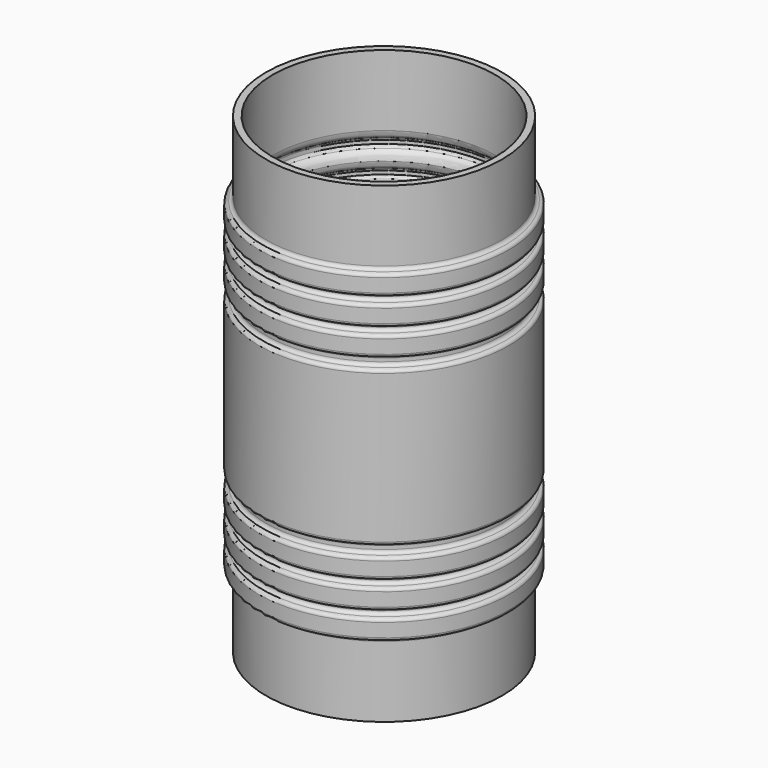
from build123d import *


# Not quite as in the source:
# - ends of sketch curves that miss each other by under 0.0002 mm in the source are joined


with BuildPart() as f1:
    # F0 (on Front) → F1 (revolve)
    with BuildSketch(Plane.XZ):
        with BuildLine():
            Line((-3.5, 2), (-3.5, 0))
            Line((-3.5, 0), (-3.3, 0))
            Line((-3.3, 0), (-3.3, 2.1))
            ThreePointArc((-3.3, 2.1), (-3.3401924262, 2.250000082), (-3.4500001641, 2.3598077159))
            ThreePointArc((-3.4500001641, 2.3598077159), (-3.4866026079, 2.396410117), (-3.5, 2.44641))
            Line((-3.5, 2.44641), (-3.5, 2.55359))
            ThreePointArc((-3.5, 2.55359), (-3.4866024829, 2.6035900995), (-3.449999801, 2.6401926553))
            ThreePointArc((-3.449999801, 2.6401926553), (-3.3401923012, 2.7500001345), (-3.3, 2.9))
            ThreePointArc((-3.3, 2.9), (-3.3401924262, 3.050000082), (-3.4500001641, 3.1598077159))
            ThreePointArc((-3.4500001641, 3.1598077159), (-3.4866026079, 3.196410117), (-3.5, 3.24641))
            Line((-3.5, 3.24641), (-3.5, 3.35359))
            ThreePointArc((-3.5, 3.35359), (-3.4866024829, 3.4035900995), (-3.449999801, 3.4401926553))
            ThreePointArc((-3.449999801, 3.4401926553), (-3.3401923012, 3.5500001345), (-3.3, 3.7))
            ThreePointArc((-3.3, 3.7), (-3.3401924262, 3.850000082), (-3.4500001641, 3.9598077159))
            ThreePointArc((-3.4500001641, 3.9598077159), (-3.4866026079, 3.996410117), (-3.5, 4.04641))
            Line((-3.5, 4.04641), (-3.5, 4.15359))
            ThreePointArc((-3.5, 4.15359), (-3.4866024829, 4.2035900995), (-3.449999801, 4.2401926553))
            ThreePointArc((-3.449999801, 4.2401926553), (-3.3401923012, 4.3500001345), (-3.3, 4.5))
            Line((-3.3, 4.5), (-3.3, 4.6))
            ThreePointArc((-3.3, 4.6), (-3.3401924262, 4.750000082), (-3.4500001641, 4.8598077159))
            ThreePointArc((-3.4500001641, 4.8598077159), (-3.4866026079, 4.896410117), (-3.5, 4.94641))
            Line((-3.5, 4.94641), (-3.5, 9.05359))
            ThreePointArc((-3.5, 9.05359), (-3.4866024829, 9.1035900995), (-3.449999801, 9.1401926553))
            ThreePointArc((-3.449999801, 9.1401926553), (-3.3401923012, 9.2500001345), (-3.3, 9.4))
            Line((-3.3, 9.4), (-3.3, 9.5))
            ThreePointArc((-3.3, 9.5), (-3.3401924262, 9.650000082), (-3.4500001641, 9.7598077159))
            ThreePointArc((-3.4500001641, 9.7598077159), (-3.4866026079, 9.796410117), (-3.5, 9.84641))
            Line((-3.5, 9.84641), (-3.5, 9.95359))
            ThreePointArc((-3.5, 9.95359), (-3.4866024829, 10.0035900995), (-3.449999801, 10.0401926553))
            ThreePointArc((-3.449999801, 10.0401926553), (-3.3401923012, 10.1500001345), (-3.3, 10.3))
            ThreePointArc((-3.3, 10.3), (-3.3401924262, 10.450000082), (-3.4500001641, 10.5598077159))
            ThreePointArc((-3.4500001641, 10.5598077159), (-3.4866026079, 10.596410117), (-3.5, 10.64641))
            Line((-3.5, 10.64641), (-3.5, 10.75359))
            ThreePointArc((-3.5, 10.75359), (-3.4866024829, 10.8035900995), (-3.449999801, 10.8401926553))
            ThreePointArc((-3.449999801, 10.8401926553), (-3.3401923012, 10.9500001345), (-3.3, 11.1))
            ThreePointArc((-3.3, 11.1), (-3.3401924262, 11.250000082), (-3.4500001641, 11.3598077159))
            ThreePointArc((-3.4500001641, 11.3598077159), (-3.4866026079, 11.396410117), (-3.5, 11.44641))
            Line((-3.5, 11.44641), (-3.5, 11.55359))
            ThreePointArc((-3.5, 11.55359), (-3.4866024829, 11.6035900995), (-3.449999801, 11.6401926553))
            ThreePointArc((-3.449999801, 11.6401926553), (-3.3401923012, 11.7500001345), (-3.3, 11.9))
            Line((-3.3, 11.9), (-3.3, 14))
            Line((-3.3, 14), (-3.5, 14))
            Line((-3.5, 14), (-3.5, 12))
            Line((-3.5, 12), (-3.5, 11.9))
            ThreePointArc((-3.5, 11.9), (-3.5292893219, 11.8292893219), (-3.6, 11.8))
            ThreePointArc((-3.6, 11.8), (-3.6707106781, 11.7707106781), (-3.7, 11.7))
            Line((-3.7, 11.7), (-3.7, 11.3))
            ThreePointArc((-3.7, 11.3), (-3.6707106781, 11.2292893219), (-3.6, 11.2))
            ThreePointArc((-3.6, 11.2), (-3.5292893219, 11.1707106781), (-3.5, 11.1))
            ThreePointArc((-3.5, 11.1), (-3.5292893219, 11.0292893219), (-3.6, 11))
            ThreePointArc((-3.6, 11), (-3.6707106781, 10.9707106781), (-3.7, 10.9))
            Line((-3.7, 10.9), (-3.7, 10.5))
            ThreePointArc((-3.7, 10.5), (-3.6707106781, 10.4292893219), (-3.6, 10.4))
            ThreePointArc((-3.6, 10.4), (-3.5292893219, 10.3707106781), (-3.5, 10.3))
            ThreePointArc((-3.5, 10.3), (-3.5292893219, 10.2292893219), (-3.6, 10.2))
            ThreePointArc((-3.6, 10.2), (-3.6707106781, 10.1707106781), (-3.7, 10.1))
            Line((-3.7, 10.1), (-3.7, 9.7))
            ThreePointArc((-3.7, 9.7), (-3.6707106781, 9.6292893219), (-3.6, 9.6))
            ThreePointArc((-3.6, 9.6), (-3.5292893219, 9.5707106781), (-3.5, 9.5))
            Line((-3.5, 9.5), (-3.5, 9.4))
            ThreePointArc((-3.5, 9.4), (-3.5292893219, 9.3292893219), (-3.6, 9.3))
            ThreePointArc((-3.6, 9.3), (-3.6707106781, 9.2707106781), (-3.7, 9.2))
            Line((-3.7, 9.2), (-3.7, 4.8))
            ThreePointArc((-3.7, 4.8), (-3.6707106781, 4.7292893219), (-3.6, 4.7))
            ThreePointArc((-3.6, 4.7), (-3.5292893219, 4.6707106781), (-3.5, 4.6))
            Line((-3.5, 4.6), (-3.5, 4.5))
            ThreePointArc((-3.5, 4.5), (-3.5292893219, 4.4292893219), (-3.6, 4.4))
            ThreePointArc((-3.6, 4.4), (-3.6707106781, 4.3707106781), (-3.7, 4.3))
            Line((-3.7, 4.3), (-3.7, 3.9))
            ThreePointArc((-3.7, 3.9), (-3.6707106781, 3.8292893219), (-3.6, 3.8))
            ThreePointArc((-3.6, 3.8), (-3.5292893219, 3.7707106781), (-3.5, 3.7))
            ThreePointArc((-3.5, 3.7), (-3.5292893219, 3.6292893219), (-3.6, 3.6))
            ThreePointArc((-3.6, 3.6), (-3.6707106781, 3.5707106781), (-3.7, 3.5))
            Line((-3.7, 3.5), (-3.7, 3.1))
            ThreePointArc((-3.7, 3.1), (-3.6707106781, 3.0292893219), (-3.6, 3))
            ThreePointArc((-3.6, 3), (-3.5292893219, 2.9707106781), (-3.5, 2.9))
            ThreePointArc((-3.5, 2.9), (-3.5292893219, 2.8292893219), (-3.6, 2.8))
            ThreePointArc((-3.6, 2.8), (-3.6707106781, 2.7707106781), (-3.7, 2.7))
            Line((-3.7, 2.7), (-3.7, 2.3))
            ThreePointArc((-3.7, 2.3), (-3.6707106781, 2.2292893219), (-3.6, 2.2))
            ThreePointArc((-3.6, 2.2), (-3.5292893219, 2.1707106781), (-3.5, 2.1))
            Line((-3.5, 2.1), (-3.5, 2))
        make_face()
    revolve(axis=Axis((0, 0, 0), (0, 0, -1)))


solid = f1.part
